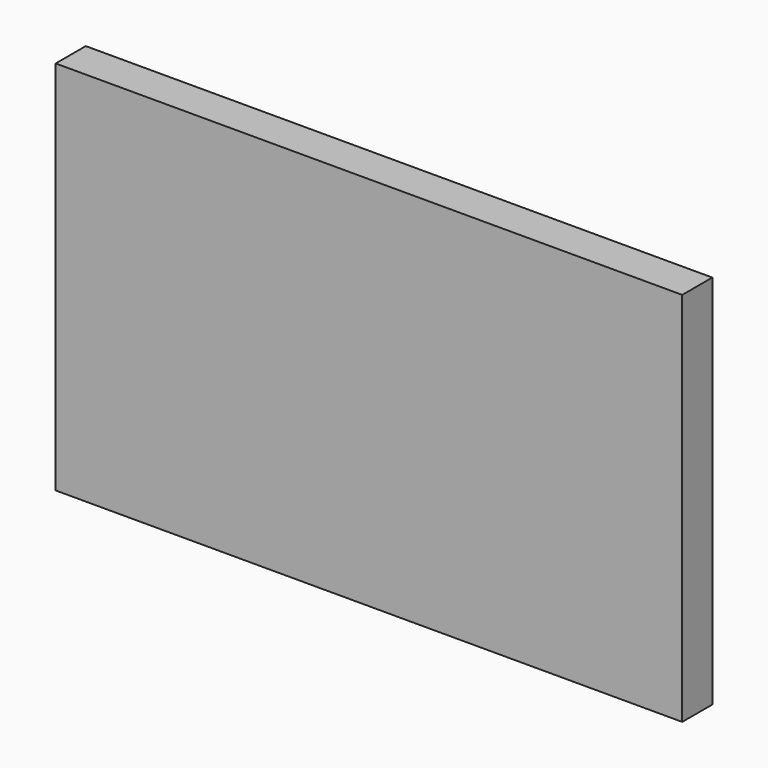
from build123d import *

# Parameters (mm, degrees)
F0_W         = 250
F0_H         = 150
F1_DEPTH     = 15
F2_R         = 25.5
F3_DEPTH     = 10
F4_TEXT_SIZE = 32.4456505532
F5_DEPTH     = 5
F6_R         = 25
F7_DEPTH     = 10


# Not quite as in the source:
# - Text() gives the source's letters only with a copy of the font that has no kerning and outlines rounded to 1/6400 em; it was checked with that copy


with BuildPart() as f1:
    # F0 (on Front) → F1 (new body)
    with BuildSketch(Plane.XZ):
        with Locations((4.5774579048, 6.5588101745)):
            Rectangle(F0_W, F0_H)
    extrude(amount=F1_DEPTH)

    # F2 (on face) → F3 (cut)
    with BuildSketch(Plane(origin=(0, 0, 0), x_dir=(-1, 0, 0), z_dir=(0, 1, 0))):
        with Locations((81.2552422285, -32.9411898255)):
            Circle(F2_R)
    extrude(amount=-F3_DEPTH, mode=Mode.SUBTRACT)

    # F4 (on face) → F5 (join)
    with BuildSketch(Plane(origin=(0, 0, 0), x_dir=(-1, 0, 0), z_dir=(0, 1, 0))):
        with Locations((-92.5106561967, 35.9894087697)):
            Text('Truffles HA', F4_TEXT_SIZE, font='Open Sans', text_align=(TextAlign.LEFT, TextAlign.BOTTOM))
    extrude(amount=F5_DEPTH)


with BuildPart() as f7:
    # F6 (on Front) → F7 (new body)
    with BuildSketch(Plane.XZ):
        with Locations((63.9801174402, 12.6323923469)):
            Circle(F6_R)
    extrude(amount=F7_DEPTH)


solid = Compound([f1.part, f7.part])
